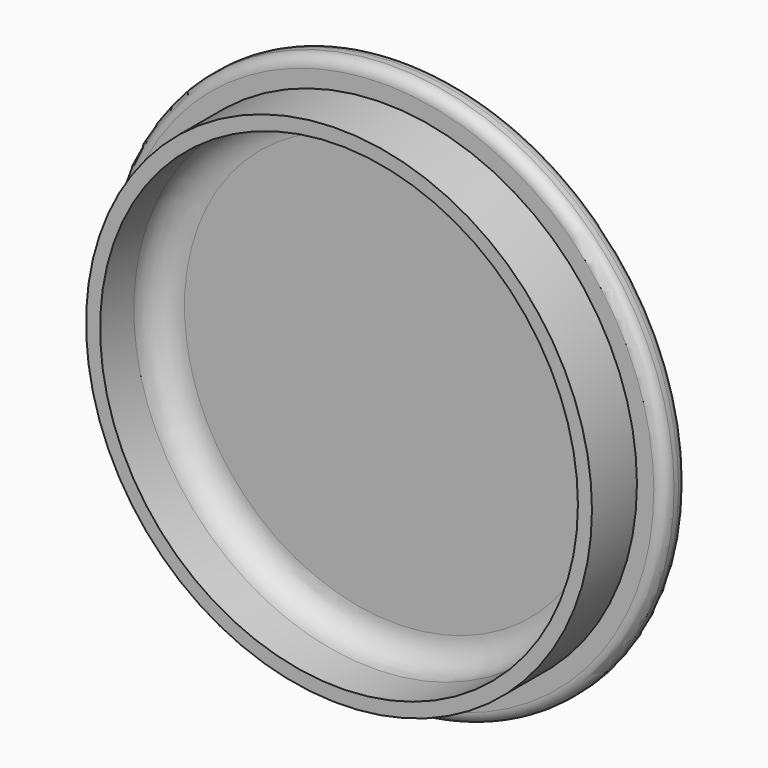
from build123d import *

# Parameters (mm, degrees)
F0_R     = 50
F1_DEPTH = 5
F3_R     = 2
F2_R     = 45
F4_DEPTH = 15
F5_T     = 2.5
F6_R     = 5


# Not quite as in the source:
# - a shell that OpenCascade refuses in one call is made with other operations: the cavity is built on its own and cut out


with BuildPart() as f1:
    # F0 (on Front) → F1 (new body)
    with BuildSketch(Plane.XZ):
        Circle(F0_R)
    extrude(amount=F1_DEPTH)

    # F3
    f3_edges = [f1.edges().sort_by_distance(p)[0] for p in [
        (-50, -5, 0),
        (-50, 0, 0),
    ]]
    fillet(f3_edges, radius=F3_R)

    # F2 (on Front) → F4 (join)
    with BuildSketch(Plane.XZ):
        Circle(F2_R)
    extrude(amount=F4_DEPTH)

    # F5: shell of thickness 2.5, made by hand


with BuildPart() as f5_core1:
    # F5_t2: copy of F1
    add(f1.part)

    # the walls: a layer under each face that stays
    f5_faces = [f5_core1.faces().sort_by_distance(p)[0] for p in [
        (-50, -2.5, 0),
        (0, 0, 0),
        (-32, -5, -32),
        (-45, -10, 0),
    ]]
    thicken(f5_faces, amount=-F5_T, mode=Mode.SUBTRACT)

    # F5_s3 → F5_t4 (revolve, cut)
    with BuildSketch(Plane.XY):
        Polygon((45.025, -5.025), (45, -2.5), (42.5, -2.5), (42.5, -5), align=None)
    revolve(axis=Axis((0, -5, 0), (0, 1, 0)), mode=Mode.SUBTRACT)


with BuildPart() as f1_1:
    add(f1.part)

    # what is left inside the walls is the cavity
    f5_cavity = [f5_core1.part.solids().sort_by_distance(p)[0] for p in [
        (0, -2.525, -14.166667),
    ]]
    add(f5_cavity, mode=Mode.SUBTRACT)

    # F6
    f6_edges = [f1_1.edges().sort_by_distance(p)[0] for p in [
        (42.5, -8.75, 0),
        (-42.5, -2.5, 0),
    ]]
    fillet(f6_edges, radius=F6_R)


solid = f1_1.part
